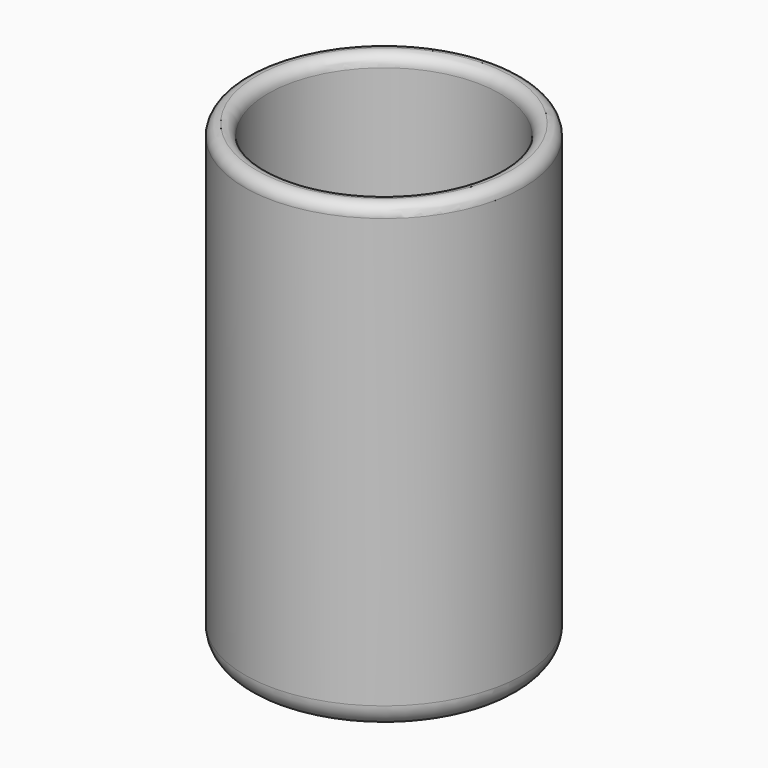
from build123d import *

# Parameters (mm, degrees)
F0_R     = 6
F0_R_2   = 2
F1_DEPTH = 20
F2_T     = -1
F3_DEPTH = 25
F4_R     = 1
F5_R     = 0.49999


# Not quite as in the source:
# - a fillet or chamfer is up to 0.001 mm smaller than in the source, because OpenCascade refuses the exact size


with BuildPart() as f1:
    # F0 (on Top) → F1 (new body)
    with BuildSketch(Plane.XY):
        Circle(F0_R)
        Circle(F0_R_2, mode=Mode.SUBTRACT)
        Circle(F0_R_2)
    extrude(amount=F1_DEPTH)

    # F2
    f2_openings = [f1.faces().sort_by_distance(p)[0] for p in [
        (0, 0, 20),
    ]]
    offset(amount=F2_T, openings=f2_openings)

    # F0 (on Top) → F3 (cut)
    with BuildSketch(Plane.XY):
        Circle(F0_R_2)
    extrude(amount=F3_DEPTH, mode=Mode.SUBTRACT)

    # F4
    f4_edges = [f1.edges().sort_by_distance(p)[0] for p in [
        (-6, 0, 0),
        (-5, 0, 1),
    ]]
    fillet(f4_edges, radius=F4_R)

    # F5 (radius 0.5 in the source; OpenCascade refuses exactly that, so slightly less here)
    f5_edges = [f1.edges().sort_by_distance(p)[0] for p in [
        (-5, 0, 20),
        (-6, 0, 20),
    ]]
    fillet(f5_edges, radius=F5_R)


solid = f1.part
